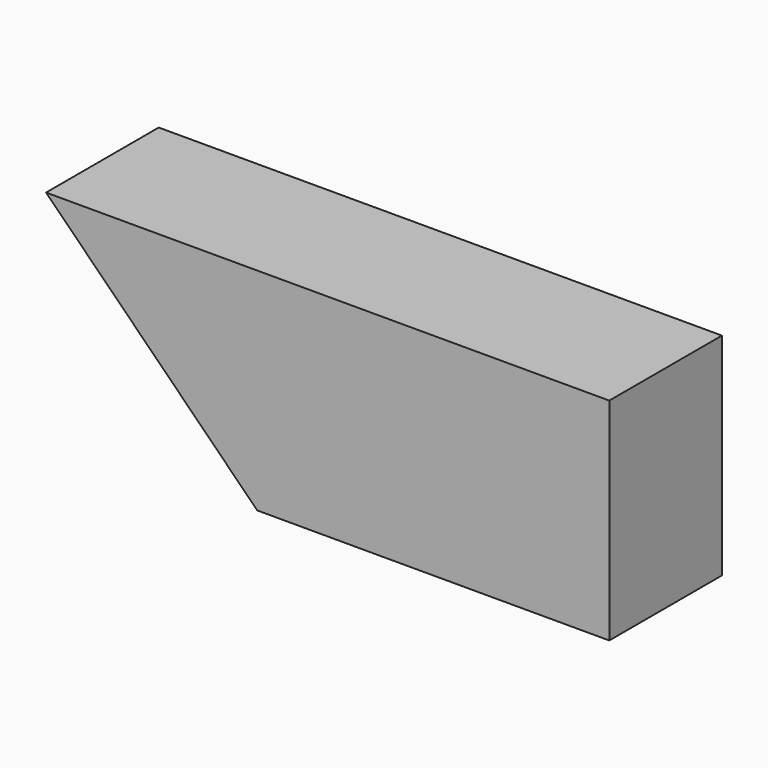
from build123d import *

# Parameters (mm, degrees)
F0_W     = 8
F0_H     = 2
F1_DEPTH = 3
F2_SIZE  = 2.99999


# Not quite as in the source:
# - a fillet or chamfer is up to 0.001 mm smaller than in the source, because OpenCascade refuses the exact size


with BuildPart() as f1:
    # F0 (on Top) → F1 (new body)
    with BuildSketch(Plane.XY):
        Rectangle(F0_W, F0_H)
    extrude(amount=F1_DEPTH)

    # F2 (size 3 in the source; OpenCascade refuses exactly that, so slightly less here)
    f2_edges = [f1.edges().sort_by_distance(p)[0] for p in [
        (-4, 0, 0),
    ]]
    chamfer(f2_edges, length=F2_SIZE)


solid = f1.part
